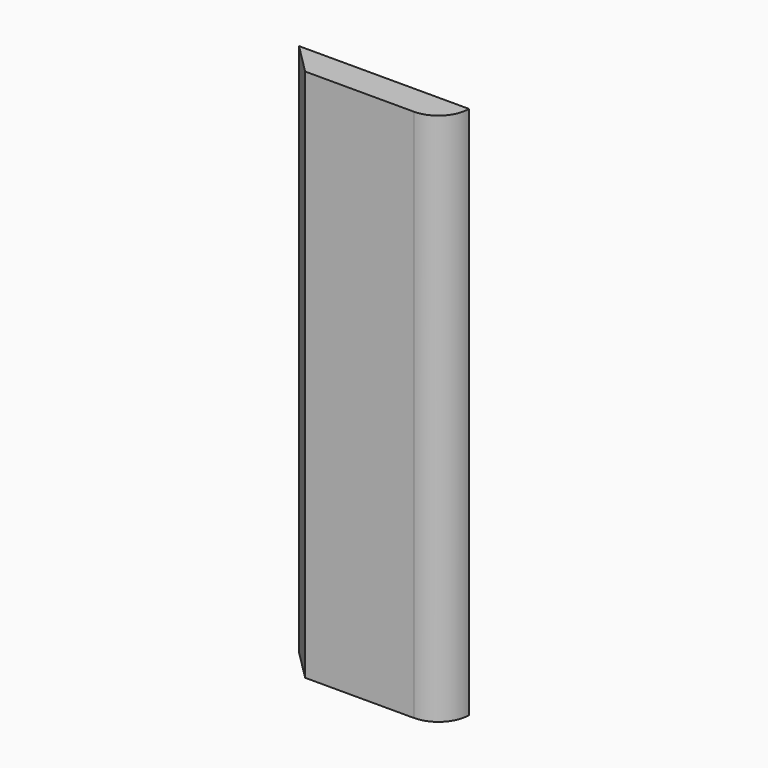
from build123d import *

# Parameters (mm, degrees)
F0_W     = 100
F0_H     = 314
F1_DEPTH = 18
F2_SIZE  = 17.99999
F3_R     = 17.99999


# Not quite as in the source:
# - a fillet or chamfer is up to 0.001 mm smaller than in the source, because OpenCascade refuses the exact size


with BuildPart() as f1:
    # F0 (on Front) → F1 (new body)
    with BuildSketch(Plane.XZ):
        Rectangle(F0_W, F0_H)
    extrude(amount=-F1_DEPTH)

    # F2 (size 18 in the source; OpenCascade refuses exactly that, so slightly less here)
    f2_edges = [f1.edges().sort_by_distance(p)[0] for p in [
        (-50, 0, 0),
    ]]
    chamfer(f2_edges, length=F2_SIZE)

    # F3 (radius 18 in the source; OpenCascade refuses exactly that, so slightly less here)
    f3_edges = [f1.edges().sort_by_distance(p)[0] for p in [
        (50, 0, 0),
    ]]
    fillet(f3_edges, radius=F3_R)


solid = f1.part
